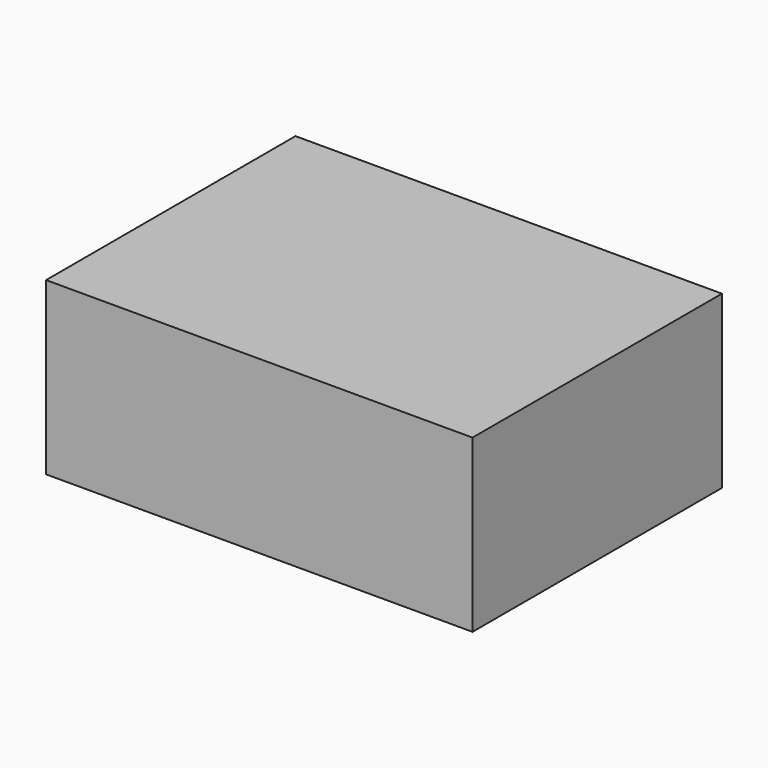
from build123d import *

# Parameters (mm, degrees)
F0_W     = 24.9305069447
F0_H     = 18.2264447212
F1_DEPTH = 9.9999997765


# Not quite as in the source:
# - the program builds the solid bodies; features that only make, move or delete a surface that nothing else refers to are left out


with BuildPart() as f1:
    # F0 (on Top) → F1 (new body)
    with BuildSketch(Plane.XY):
        with Locations((133.3001405001, 21.3852450252)):
            Rectangle(F0_W, F0_H)
    extrude(amount=F1_DEPTH)


solid = f1.part
